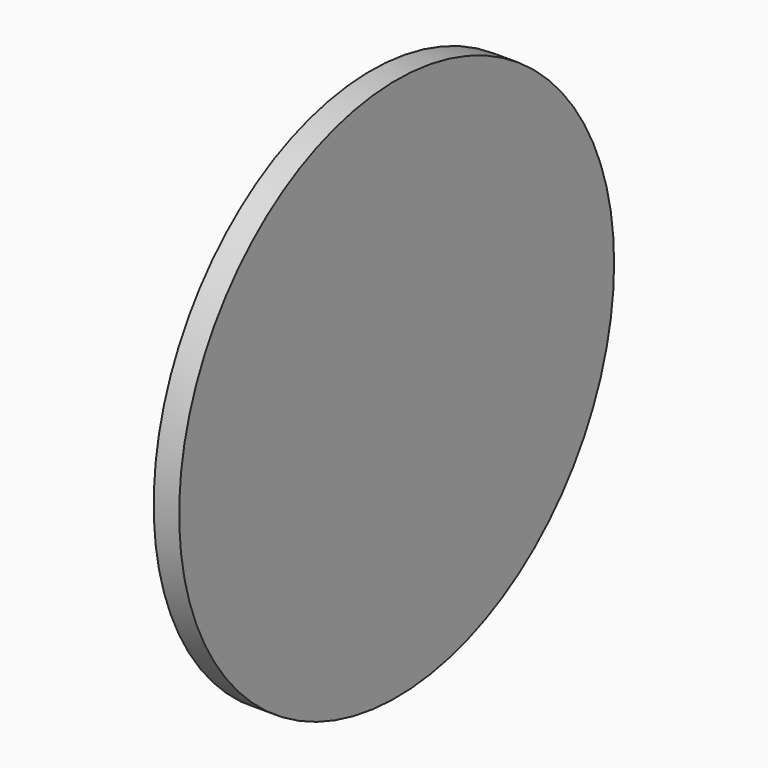
from build123d import *

# Parameters (mm, degrees)
F0_R     = 50.8
F1_DEPTH = 4.7625
F2_R     = 3.175
F3_DEPTH = 0.02286


# Not quite as in the source:
# - a length typed as a fraction of an inch, garbled in the dataset ("3 / 203.2 mm" for 3/8 in), is restored


with BuildPart() as f1:
    # F0 (on Right) → F1 (new body)
    with BuildSketch(Plane.YZ):
        Circle(F0_R)
    extrude(amount=F1_DEPTH)

    # F2 (on Right) → F3 (cut)
    with BuildSketch(Plane.YZ):
        Circle(F2_R)
    extrude(amount=F3_DEPTH, mode=Mode.SUBTRACT)


solid = f1.part
